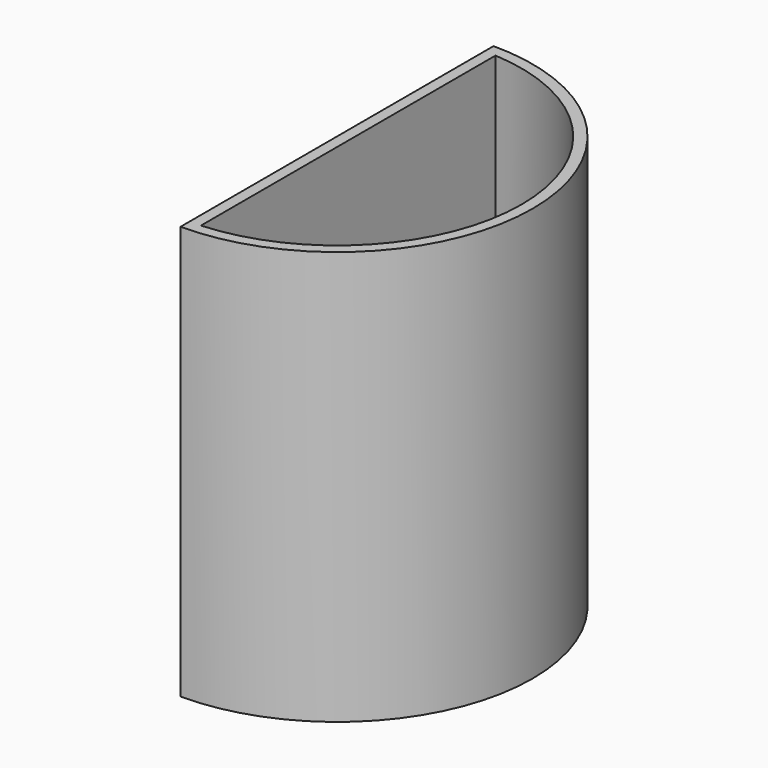
from build123d import *

# Parameters (mm, degrees)
F1_DEPTH     = 93.98
F2_T         = -2.54
F3_TEXT_SIZE = 9.7367554131
F4_DEPTH     = 1


# Not quite as in the source:
# - Text() gives the source's letters only with a copy of the font that has no kerning and outlines rounded to 1/6400 em; it was checked with that copy


with BuildPart() as f1:
    # F0 (on Top) → F1 (new body)
    with BuildSketch(Plane.XY):
        with BuildLine():
            ThreePointArc((0, -44.45), (44.45, 0), (0, 44.45))
            Line((0, 44.45), (0, -44.45))
        make_face()
    extrude(amount=F1_DEPTH)

    # F2
    f2_openings = [f1.faces().sort_by_distance(p)[0] for p in [
        (18.865166, 0, 93.98),
    ]]
    offset(amount=F2_T, openings=f2_openings)

    # F3 (on face) → F4 (join)
    with BuildSketch(Plane.XY.offset(2.54)):
        with Locations(Location((22.2504638975, -25.4), (0, 0, 90))):
            Text('Day Dream', F3_TEXT_SIZE, font='Open Sans', text_align=(TextAlign.LEFT, TextAlign.BOTTOM))
    extrude(amount=F4_DEPTH)


solid = f1.part
